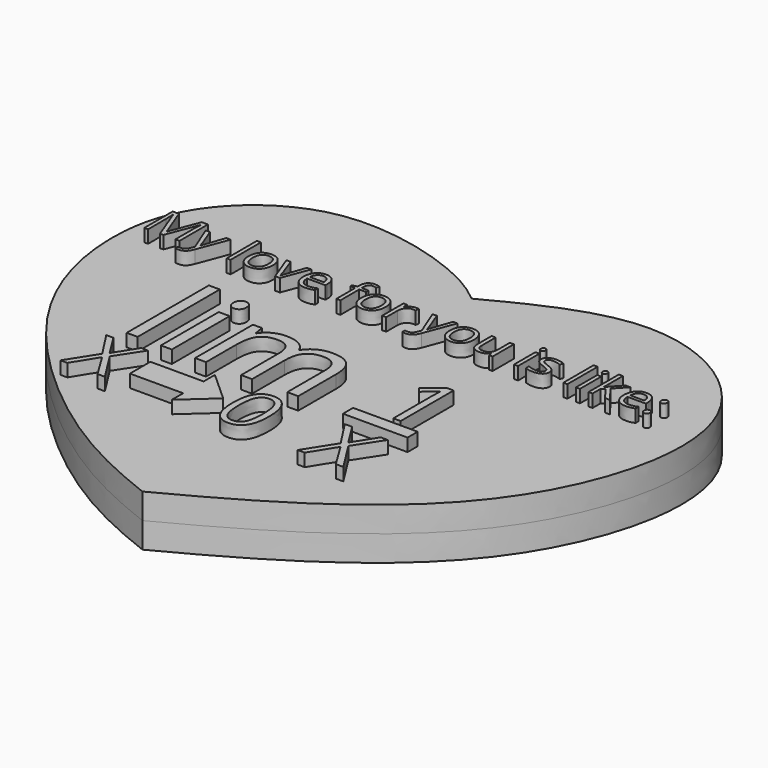
from build123d import *

# Parameters (mm, degrees)
F1_DEPTH       = 4
F2_SCALE       = 0.5
F3_W           = 5.0472486764
F3_H           = 0.9896568954
F3_TEXT_SIZE   = 3.8923521362
F3_TEXT_SIZE_2 = 10.5645427534
F3_TEXT_SIZE_3 = 6.0894386299
F3_TEXT_SIZE_4 = 7.24801812
F3_TEXT_SIZE_5 = 6.2683643487
F4_DEPTH       = 3


# Not quite as in the source:
# - Text() gives the source's letters only with a copy of the font that has no kerning and outlines rounded to 1/6400 em; it was checked with that copy


with BuildPart() as f1:
    # F0 (on Top) → F1 (new body, symmetric)
    with BuildSketch(Plane.XY):
        with BuildLine():
            add(Edge.make_bspline(
                [(49.6034175158, 70.3383758664), (57.4255755938, 74.4701894092), (72.777071302, 82.1686280864), (98.5809075936, 66.4625184016), (89.6533310415, 28.6744955736), (66.9245487128, 14.178657317), (50.0742010772, 5.4191295058)],
                knots=[0, 0, 0, 0, 0.2245214689, 0.4410611027, 0.6922062561, 1, 1, 1, 1], degree=3))
            add(Edge.make_bspline(
                [(49.6034175158, 70.3383758664), (47.4339338141, 72.2192165566), (41.0433747036, 76.0012562734), (22.277013048, 80.0594704424), (7.7702176976, 69.6318815381), (3.9007087353, 55.4213262189), (8.818104806, 34.6134665552), (31.3463892668, 13.6516026811), (43.7721535607, 7.8800658319), (50.0742010772, 5.4191295058)],
                knots=[0, 0, 0, 0, 0.106242303, 0.2507252939, 0.3862136345, 0.5102499506, 0.6625335349, 0.8471651701, 1, 1, 1, 1], degree=3))
        make_face()
    extrude(amount=F1_DEPTH, both=True)


with BuildPart() as f1_1:
    # F2: moved
    add(f1.part.scale(F2_SCALE))

    # F3 (on Top) → F4 (join)
    with BuildSketch(Plane.XY):
        Polygon((20.0663190335, 14.905732125), (15.905328095, 14.905732125), (15.905328095, 12.9084568471), (20.0663190335, 12.9084568471), (20.0663190335, 11.8020772934), (22.3964750767, 13.9070944861), (20.0663190335, 16.0121116787), align=None)
        with Locations((31.8987322971, 17.3831116408)):
            Rectangle(F3_W, F3_H)
        with Locations((4.1777360804, 28.4927999253)):
            Text('My love for you is like:', F3_TEXT_SIZE, font='Open Sans', text_align=(TextAlign.LEFT, TextAlign.BOTTOM))
        with Locations((11.4787481725, 16.9918911419)):
            Text('lim', F3_TEXT_SIZE_2, font='Open Sans', text_align=(TextAlign.LEFT, TextAlign.BOTTOM))
        with Locations((11.4807039499, 11.6277158652)):
            Text('X     0', F3_TEXT_SIZE_3, font='Open Sans', text_align=(TextAlign.LEFT, TextAlign.BOTTOM))
        with Locations((30.1989745349, 18.3304770463)):
            Text('1', F3_TEXT_SIZE_4, font='Open Sans', text_align=(TextAlign.LEFT, TextAlign.BOTTOM))
        with Locations((30.1904100925, 11.412177628)):
            Text('X', F3_TEXT_SIZE_5, font='Open Sans', text_align=(TextAlign.LEFT, TextAlign.BOTTOM))
    extrude(amount=F4_DEPTH)


solid = f1_1.part
